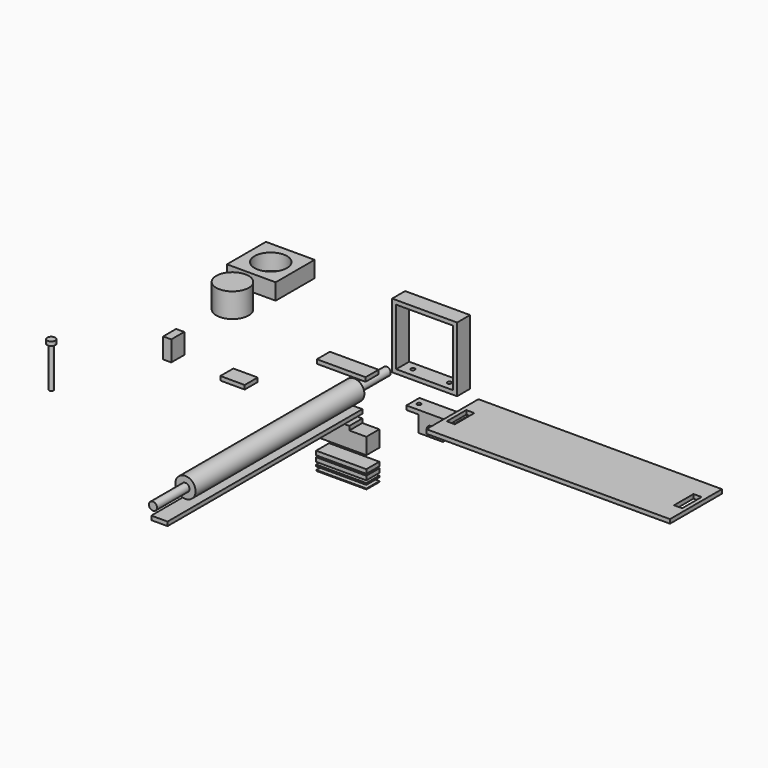
from build123d import *

# Parameters (mm, degrees)
F0_R      = 5
F1_DEPTH  = 20
F0_W      = 60
F0_H      = 5
F0_W_2    = 80
F0_H_2    = 80
F0_W_3    = 70
F0_H_3    = 70
F0_W_4    = 61.861140081
F0_H_4    = 1
F0_H_5    = 2
F0_R_2    = 12.5
F2_DEPTH  = 260
F3_R      = 5
F4_DEPTH  = 50
F5_DEPTH  = 300
F6_R      = 2.5
F7_DEPTH  = 25
F9_R      = 2.5
F8_R      = 2.5
F10_DEPTH = 25
F14_R     = 5
F15_DEPTH = 50
F16_W     = 300
F16_H     = 5
F17_DEPTH = 80
F19_R     = 20
F20_DEPTH = 30
F19_W     = 60
F19_H     = 60
F21_DEPTH = 20
F18_W     = 10
F18_H     = 30
F22_DEPTH = 129.4251411048
F18_H_2   = 20
F23_DEPTH = 25
F18_W_2   = 30
F24_DEPTH = 5
F13_R     = 2.5
F25_DEPTH = 5
F26_R     = 5
F27_DEPTH = 5
F28_R     = 2.5
F29_DEPTH = 50


# Not quite as in the source:
# - a feature of the source that left no trace in its solid (it failed there, or was rolled back) is left out
# - a feature names something its author has since deleted; it is built from what else it names


with BuildPart() as f1:
    # F0 (on Front) → F1 (new body)
    with BuildSketch(Plane.XZ):
        Polygon((95.2936565876, -7.5), (110.2936565876, -7.5), (125.2936565876, -7.5), (125.2936565876, 12.5), (140.2936565876, 12.5), (140.2936565876, 17.5), (110.2936565876, 17.5), (80.2936565876, 17.5), (80.2936565876, 12.5), (95.2936565876, 12.5), align=None)
        with Locations((110.2936565876, 0)):
            Circle(F0_R, mode=Mode.SUBTRACT)
    extrude(amount=F1_DEPTH)

    # F9 (on face) + F8 (on face) → F10 (cut)
    with BuildSketch(Plane(origin=(0, 0, 12.5), x_dir=(1, 0, 0), z_dir=(0, 0, -1))):
        with Locations((87.7936565876, 10)):
            Circle(F9_R)
    with BuildSketch(Plane(origin=(0, 0, 12.5), x_dir=(1, 0, 0), z_dir=(0, 0, -1))):
        with Locations((132.7936565876, 10)):
            Circle(F8_R)
    extrude(amount=-F10_DEPTH, mode=Mode.SUBTRACT)


with BuildPart() as f1b:
    # F0 (on Front) → F1, piece 2 (new body)
    with BuildSketch(Plane.XZ):
        with Locations((0, 29.2427036911)):
            Rectangle(F0_W, F0_H)
    extrude(amount=F1_DEPTH)


with BuildPart() as f1c:
    # F0 (on Front) → F1, piece 3 (new body)
    with BuildSketch(Plane.XZ):
        Polygon((10, -27.5771580637), (0, -27.5771580637), (-10, -27.5771580637), (-10, -32.5771580637), (-10.9305700405, -32.5771580637), (-30.9305700405, -32.5771580637), (-30.9305700405, -52.5771580637), (0, -52.5771580637), (30.9305700405, -52.5771580637), (30.9305700405, -32.5771580637), (10.9305700405, -32.5771580637), (10, -32.5771580637), align=None)
    extrude(amount=F1_DEPTH)

    # F6 (on face) → F7 (cut)
    with BuildSketch(Plane.XY.offset(-32.5771580637)):
        with Locations((-20, -10)):
            Circle(F6_R)
    extrude(amount=-F7_DEPTH, mode=Mode.SUBTRACT)


with BuildPart() as f1d:
    # F0 (on Front) → F1, piece 4 (new body)
    with BuildSketch(Plane.XZ):
        with Locations((102.7326732874, 87.7068325877)):
            Rectangle(F0_W_2, F0_H_2)
        with Locations((102.7326732874, 87.7068325877)):
            Rectangle(F0_W_3, F0_H_3, mode=Mode.SUBTRACT)
    extrude(amount=F1_DEPTH)

    # F13 (on face) → F25 (cut, through all)
    with BuildSketch(Plane(origin=(0, 0, 47.7068325877), x_dir=(1, 0, 0), z_dir=(0, 0, -1))):
        with Locations((125.2326732874, 10)):
            Circle(F13_R)
        with Locations((80.2326732874, 10)):
            Circle(F13_R)
    extrude(amount=-F25_DEPTH, mode=Mode.SUBTRACT)


with BuildPart() as f1e:
    # F0 (on Front) → F1, piece 5 (new body)
    with BuildSketch(Plane.XZ):
        with Locations((0, -77.355325222)):
            Rectangle(F0_W_4, F0_H)
    extrude(amount=F1_DEPTH)


with BuildPart() as f1f:
    # F0 (on Front) → F1, piece 6 (new body)
    with BuildSketch(Plane.XZ):
        with Locations((0.1928325291, -89.1451310813)):
            Rectangle(F0_W_4, F0_H_4)
    extrude(amount=F1_DEPTH)


with BuildPart() as f1g:
    # F0 (on Front) → F1, piece 7 (new body)
    with BuildSketch(Plane.XZ):
        with Locations((0, -83.756296128)):
            Rectangle(F0_W_4, F0_H_5)
    extrude(amount=F1_DEPTH)


with BuildPart() as f1h:
    # F0 (on Front) → F1, piece 8 (new body)
    with BuildSketch(Plane.XZ):
        with Locations((0, -70.2389810979)):
            Rectangle(F0_W_4, F0_H)
    extrude(amount=F1_DEPTH)


with BuildPart() as f2:
    # F0 (on Front) → F2 (new body)
    with BuildSketch(Plane.XZ):
        Circle(F0_R_2)
    extrude(amount=F2_DEPTH)

    # F3 (on face) → F4 (join)
    with BuildSketch(Plane.XZ.offset(260)):
        Circle(F3_R)
    extrude(amount=F4_DEPTH)

    # F14 (on face) → F15 (join)
    with BuildSketch(Plane(origin=(0, 0, 0), x_dir=(-1, 0, 0), z_dir=(0, 1, 0))):
        Circle(F14_R)
    extrude(amount=F15_DEPTH)


with BuildPart() as f5:
    # F0 (on Front) → F5 (new body)
    with BuildSketch(Plane.XZ):
        Polygon((-10, -22.5167013705), (0, -22.5167013705), (10, -22.5167013705), (10, -17.5167013705), (0, -17.5167013705), (-10, -17.5167013705), align=None)
    extrude(amount=F5_DEPTH)


with BuildPart() as f17:
    # F16 (on Front) → F17 (new body)
    with BuildSketch(Plane.XZ):
        with Locations((303.0256081372, 37.2790100235)):
            Rectangle(F16_W, F16_H)
    extrude(amount=F17_DEPTH)

    # F18 (on face) → F22 (cut, through all)
    with BuildSketch(Plane.XY.offset(39.7790100235)):
        with Locations((163.0256081372, -40)):
            Rectangle(F18_W, F18_H)
        with Locations((443.0256081372, -40)):
            Rectangle(F18_W, F18_H)
    extrude(amount=-F22_DEPTH, mode=Mode.SUBTRACT)


with BuildPart() as f20:
    # F19 (on Top) → F20 (new body)
    with BuildSketch(Plane.XY):
        with Locations((-196.2528675795, 57.794149965)):
            Circle(F19_R)
    extrude(amount=F20_DEPTH)


with BuildPart() as f21:
    # F19 (on Top) → F21 (new body)
    with BuildSketch(Plane.XY):
        with Locations((-205.1943850517, 127.9719012976)):
            Rectangle(F19_W, F19_H)
        with Locations((-205.1943850517, 127.9719012976)):
            Circle(F19_R, mode=Mode.SUBTRACT)
    extrude(amount=F21_DEPTH)


with BuildPart() as f23:
    # F18 (on face) → F23 (new body)
    with BuildSketch(Plane.XY.offset(39.7790100235)):
        with Locations((-130.5344802141, -114.8494374752)):
            Rectangle(F18_W, F18_H_2)
    extrude(amount=F23_DEPTH)


with BuildPart() as f24:
    # F18 (on face) → F24 (new body)
    with BuildSketch(Plane.XY.offset(39.7790100235)):
        with Locations((-50.0688782334, -114.8494374752)):
            Rectangle(F18_W_2, F18_H_2)
    extrude(amount=F24_DEPTH)


with BuildPart() as f27:
    # F26 (on Top) → F27 (new body)
    with BuildSketch(Plane.XY):
        with Locations((-287.8777384163, -106.7102653366)):
            Circle(F26_R)
    extrude(amount=F27_DEPTH)

    # F28 (on face) → F29 (join)
    with BuildSketch(Plane.XY):
        with Locations((-287.7346277237, -106.8533882499)):
            Circle(F28_R)
    extrude(amount=-F29_DEPTH)


solid = Compound([f1.part, f1b.part, f1c.part, f1d.part, f1e.part, f1f.part, f1g.part, f1h.part, f2.part, f5.part, f17.part, f20.part, f21.part, f23.part, f24.part, f27.part])
